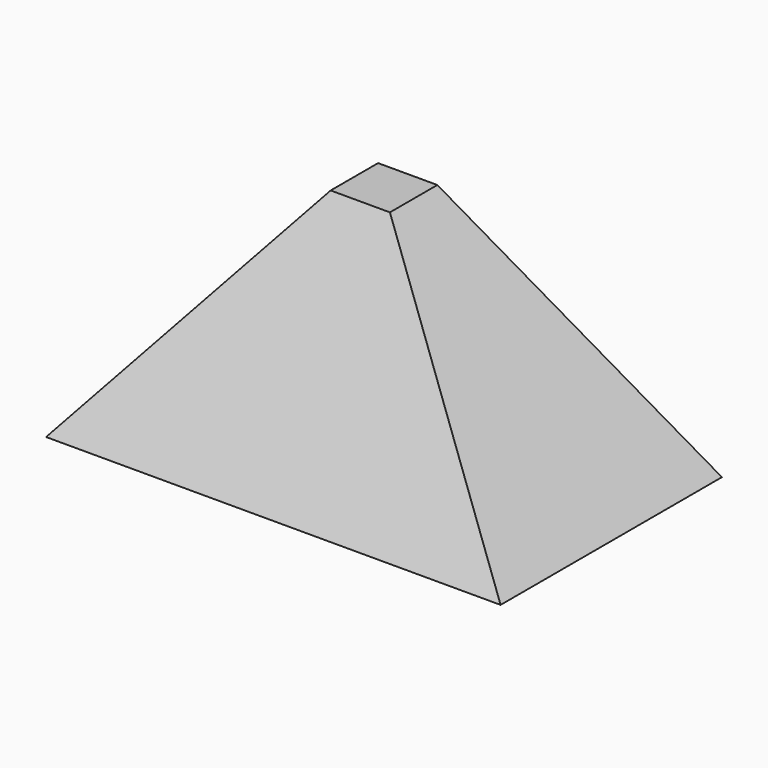
from build123d import *

# Parameters (mm, degrees)
F0_W       = 23
F0_H       = 14
F1_DEPTH   = 12
F2_SIZE2   = 11.99999
F2_SIZE    = 9.99999
F3_SIZE2   = 5.49999
F3_SIZE    = 11.99999
F3_2_SIZE2 = 5.49999
F3_2_SIZE  = 11.99999


# Not quite as in the source:
# - a fillet or chamfer is up to 0.001 mm smaller than in the source, because OpenCascade refuses the exact size


with BuildPart() as f1:
    # F0 (on Top) → F1 (new body)
    with BuildSketch(Plane.XY):
        Rectangle(F0_W, F0_H)
    extrude(amount=F1_DEPTH)

    # F2 (size 10 and 12 in the source; OpenCascade refuses exactly that, so slightly less here)
    f2_edges = [f1.edges().sort_by_distance(p)[0] for p in [
        (-11.5, 0, 12),
        (11.5, 0, 12),
    ]]
    f2_side = f1.faces().sort_by_distance((0, 0, 12))[0]
    chamfer(f2_edges, length=F2_SIZE, length2=F2_SIZE2, reference=f2_side)

    # F3 (size 12 and 5.5 in the source; OpenCascade refuses exactly that, so slightly less here)
    f3_edges = [f1.edges().sort_by_distance(p)[0] for p in [
        (0, -7, 12),
    ]]
    f3_side = f1.faces().sort_by_distance((0, -7, 4.461541))[0]
    chamfer(f3_edges, length=F3_SIZE, length2=F3_SIZE2, reference=f3_side)

    # F3#2 (size 12 and 5.5 in the source; OpenCascade refuses exactly that, so slightly less here)
    f3_2_edges = [f1.edges().sort_by_distance(p)[0] for p in [
        (0, 7, 12),
    ]]
    f3_2_side = f1.faces().sort_by_distance((0, 7, 4.461541))[0]
    chamfer(f3_2_edges, length=F3_2_SIZE, length2=F3_2_SIZE2, reference=f3_2_side)


solid = f1.part
